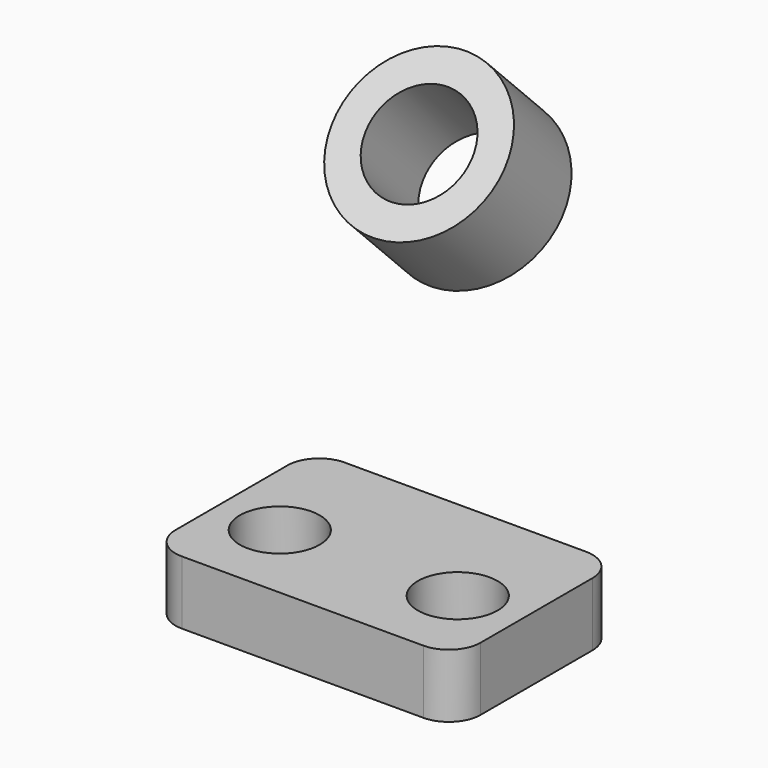
from build123d import *

# Parameters (mm, degrees)
F0_W     = 96
F0_H     = 64
F1_DEPTH = 20
F2_R     = 10
F3_R     = 12.5650724874
F4_DEPTH = 25
F8_R     = 26
F8_R_2   = 16
F9_DEPTH = 32


with BuildPart() as f1:
    # F0 (on Top) → F1 (new body)
    with BuildSketch(Plane.XY):
        Rectangle(F0_W, F0_H)
    extrude(amount=F1_DEPTH)

    # F2
    f2_edges = [f1.edges().sort_by_distance(p)[0] for p in [
        (-48, -32, 10),
        (48, -32, 10),
        (48, 32, 10),
        (-48, 32, 10),
    ]]
    fillet(f2_edges, radius=F2_R)

    # F3 (on Top) → F4 (cut)
    with BuildSketch(Plane.XY):
        with Locations((28, -6)):
            Circle(F3_R)
        with Locations((-28, -6)):
            Circle(F3_R)
    extrude(amount=F4_DEPTH, mode=Mode.SUBTRACT)


with BuildPart() as f9:
    # F8 (on offset) → F9 (new body)
    with BuildSketch(Plane(origin=(0, -57.0549957007, 57.0549957007), x_dir=(-1, 0, 0), z_dir=(0, 0.7071067812, -0.7071067812))):
        with Locations((0, 100.2076724347)):
            Circle(F8_R)
        with Locations((0, 100.2076724347)):
            Circle(F8_R_2, mode=Mode.SUBTRACT)
    extrude(amount=F9_DEPTH)


solid = Compound([f1.part, f9.part])
